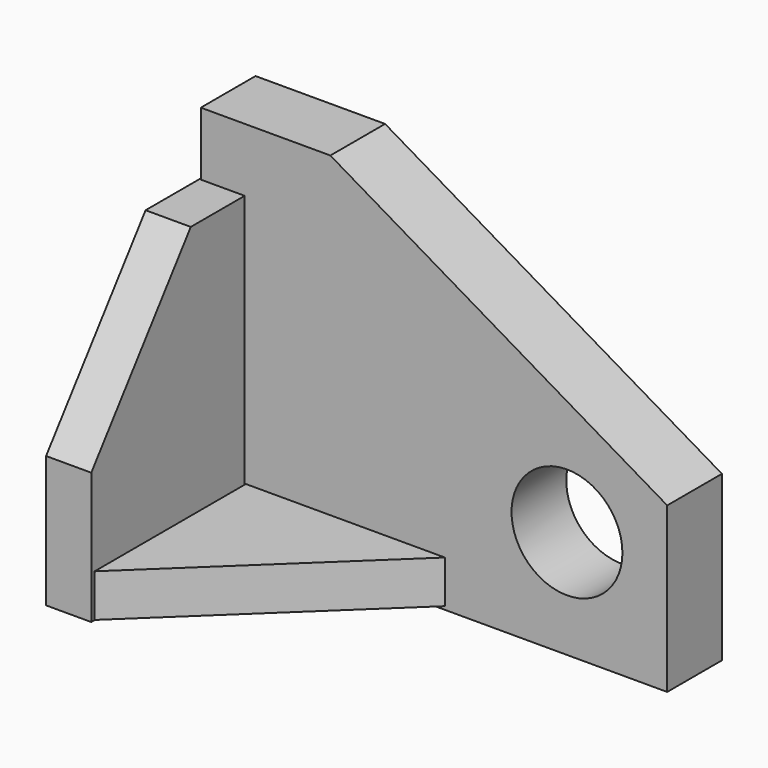
from build123d import *

# Parameters (mm, degrees)
F0_R        = 13.5872580749
F1_DEPTH    = 16.764
F2_W        = 11.076066643
F2_H        = 72.8688556701
F3_DEPTH    = 63.754
F4_SIZE2    = 40.64
F4_SIZE     = 30.48
F5_W        = 49.8422943056
F5_H        = 10.4931145906
F6_DEPTH    = 64.008
F7_T4_DEPTH = 271.9527686037


# Not quite as in the source:
# - a fillet or chamfer that OpenCascade refuses, or shapes differently, is made with other operations: its cross-section is extruded or revolved along the edge and cut away or added


with BuildPart() as f1:
    # F0 (on Front) → F1 (new body)
    with BuildSketch(Plane.XZ):
        Polygon((-29.1315091585, 37.5352683077), (-60.8815091585, 37.5352683077), (-60.8815091585, -51.3647316923), (53.4184908415, -51.3647316923), (53.4184908415, -11.1139282757), align=None)
        with Locations((28.8560632616, -24.9211471528)):
            Circle(F0_R, mode=Mode.SUBTRACT)
    extrude(amount=F1_DEPTH)

    # F2 (on Front) → F3 (join)
    with BuildSketch(Plane.XZ):
        with Locations((-55.6718055159, -14.4280334935)):
            Rectangle(F2_W, F2_H)
    extrude(amount=F3_DEPTH)

    # F4
    f4_edges = [f1.edges().sort_by_distance(p)[0] for p in [
        (-55.671806, -63.754, 22.006394),
    ]]
    f4_side = f1.faces().sort_by_distance((-55.728042, -39.925416, 22.006394))[0]
    chamfer(f4_edges, length=F4_SIZE, length2=F4_SIZE2, reference=f4_side)

    # F5 (on Front) → F6 (join)
    with BuildSketch(Plane.XZ):
        with Locations((-24.9211471528, -45.3244261444)):
            Rectangle(F5_W, F5_H)
    extrude(amount=F6_DEPTH)

    # F7: chamfer of 48.26 x 50.8 on 1 edges, made by hand


with BuildPart() as f7_tool2:
    # F7_s3 → F7_t4 (new body)
    with BuildSketch(Plane.XY.offset(-181.3008104462)):
        Polygon((0, -15.748), (-50.8, -64.008), (0, -64.008), align=None)
    extrude(amount=F7_T4_DEPTH)

    split(bisect_by=Plane.XZ.offset(16.764), keep=Keep.TOP)

    split(bisect_by=Plane.YZ.offset(-49.8422943056), keep=Keep.TOP)


with BuildPart() as f1_1:
    add(f1.part)

    # F7_t1: cut F7_tool2
    add(f7_tool2.part, mode=Mode.SUBTRACT)


solid = f1_1.part
